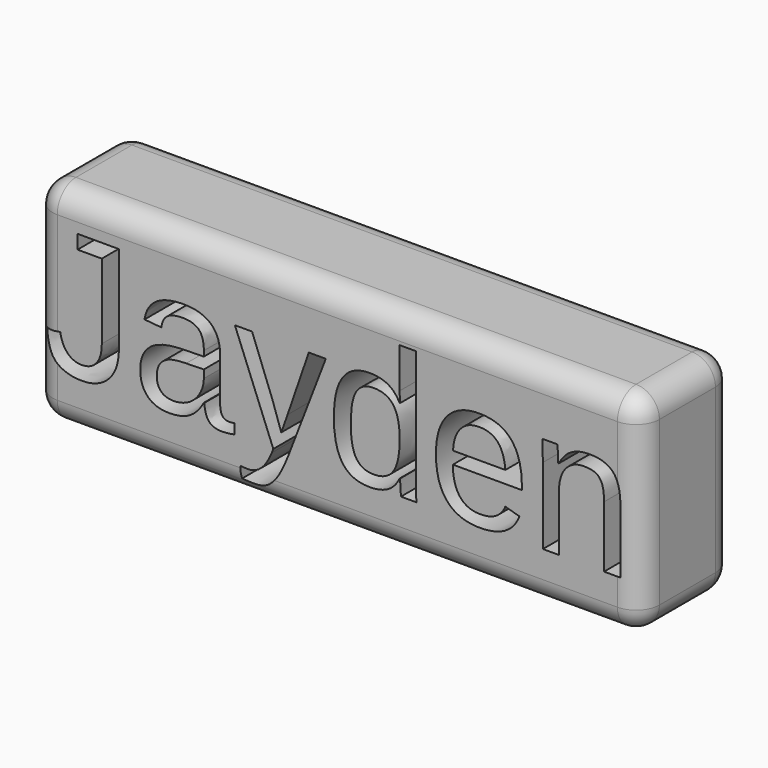
from build123d import *

# Parameters (mm, degrees)
F0_W         = 130
F0_H         = 45
F1_DEPTH     = 25
F2_TEXT_SIZE = 39.2966263462
F3_DEPTH     = 25
F4_T1_DEPTH  = 15
F4_T3_DEPTH  = 35
F4_T5_DEPTH  = 120
F4_S9_W      = 5
F4_S9_H      = 5
F4_T10_DEPTH = 5
F4_S15_W     = 5
F4_S15_H     = 5
F4_T16_DEPTH = 5
F4_S21_W     = 5
F4_S21_H     = 5
F4_T22_DEPTH = 5
F4_S27_W     = 5
F4_S27_H     = 5
F4_T28_DEPTH = 5
F4_S33_W     = 5
F4_S33_H     = 5
F4_T34_DEPTH = 5
F4_S39_W     = 5
F4_S39_H     = 5
F4_T40_DEPTH = 5
F4_S45_W     = 5
F4_S45_H     = 5
F4_T46_DEPTH = 5
F4_S51_W     = 5
F4_S51_H     = 5
F4_T52_DEPTH = 5


# Not quite as in the source:
# - a fillet or chamfer that OpenCascade refuses, or shapes differently, is made with other operations: its cross-section is extruded or revolved along the edge and cut away or added
# - Text() gives the source's letters only with a copy of the font that has no kerning and outlines rounded to 1/6400 em; it was checked with that copy


with BuildPart() as f1:
    # F0 (on Front) → F1 (new body)
    with BuildSketch(Plane.XZ):
        with Locations((65, 22.5)):
            Rectangle(F0_W, F0_H)
    extrude(amount=-F1_DEPTH)

    # F2 (on face) → F3 (cut)
    with BuildSketch(Plane.XZ):
        with Locations((1.4560963027, 10.7717518695)):
            Text('Jayden', F2_TEXT_SIZE, font='Arimo', text_align=(TextAlign.LEFT, TextAlign.BOTTOM))
    extrude(amount=-F3_DEPTH, mode=Mode.SUBTRACT)

    # F4: fillet of radius 5 on 12 edges, made by hand

    # F4_s2 → F4_t1 (cut)
    with BuildSketch(Plane.XZ.offset(-20)):
        with BuildLine():
            ThreePointArc((125, 0), (128.5355339059, 1.4644660941), (130, 5))
            Line((130, 5), (130, 0))
            Line((130, 0), (125, 0))
        make_face()
        with BuildLine():
            ThreePointArc((125, 45), (128.5355339059, 43.5355339059), (130, 40))
            Line((130, 40), (130, 45))
            Line((130, 45), (125, 45))
        make_face()
        with BuildLine():
            ThreePointArc((0, 40), (1.4644660941, 43.5355339059), (5, 45))
            Line((5, 45), (0, 45))
            Line((0, 45), (0, 40))
        make_face()
        with BuildLine():
            ThreePointArc((0, 5), (1.4644660941, 1.4644660941), (5, 0))
            Line((5, 0), (0, 0))
            Line((0, 0), (0, 5))
        make_face()
    extrude(amount=F4_T1_DEPTH, mode=Mode.SUBTRACT)

    # F4_s4 → F4_t3 (cut)
    with BuildSketch(Plane.XY.offset(5)):
        with BuildLine():
            ThreePointArc((125, 0), (128.5355339059, 1.4644660941), (130, 5))
            Line((130, 5), (130, 0))
            Line((130, 0), (125, 0))
        make_face()
        with BuildLine():
            ThreePointArc((125, 25), (128.5355339059, 23.5355339059), (130, 20))
            Line((130, 20), (130, 25))
            Line((130, 25), (125, 25))
        make_face()
        with BuildLine():
            ThreePointArc((0, 5), (1.4644660941, 1.4644660941), (5, 0))
            Line((5, 0), (0, 0))
            Line((0, 0), (0, 5))
        make_face()
        with BuildLine():
            ThreePointArc((0, 20), (1.4644660941, 23.5355339059), (5, 25))
            Line((5, 25), (0, 25))
            Line((0, 25), (0, 20))
        make_face()
    extrude(amount=F4_T3_DEPTH, mode=Mode.SUBTRACT)

    # F4_s6 → F4_t5 (cut)
    with BuildSketch(Plane.YZ.offset(5)):
        with BuildLine():
            ThreePointArc((5, 45), (1.4644660941, 43.5355339059), (0, 40))
            Line((0, 40), (0, 45))
            Line((0, 45), (5, 45))
        make_face()
        with BuildLine():
            ThreePointArc((20, 45), (23.5355339059, 43.5355339059), (25, 40))
            Line((25, 40), (25, 45))
            Line((25, 45), (20, 45))
        make_face()
        with BuildLine():
            ThreePointArc((5, 0), (1.4644660941, 1.4644660941), (0, 5))
            Line((0, 5), (0, 0))
            Line((0, 0), (5, 0))
        make_face()
        with BuildLine():
            ThreePointArc((20, 0), (23.5355339059, 1.4644660941), (25, 5))
            Line((25, 5), (25, 0))
            Line((25, 0), (20, 0))
        make_face()
    extrude(amount=F4_T5_DEPTH, mode=Mode.SUBTRACT)


with BuildPart() as f4_tool8:
    # F4_s9 → F4_t10 (new body)
    with BuildSketch(Plane.XY.offset(5)):
        with Locations((127.5, 2.5)):
            Rectangle(F4_S9_W, F4_S9_H)
    extrude(amount=-F4_T10_DEPTH)

    # F4_s11 → F4_t12 (revolve, cut)
    with BuildSketch(Plane(origin=(125, 5, 5), x_dir=(-0.7071067812, 0.7071067812, 0), z_dir=(-0.7071067812, -0.7071067812, 0))):
        with BuildLine():
            ThreePointArc((0, -5), (5, 0), (0, 5))
            Line((0, 5), (0, -5))
        make_face()
    revolve(axis=Axis((125, 5, 5), (0, 0, -1)), mode=Mode.SUBTRACT)


with BuildPart() as f1_1:
    add(f1.part)

    # F4_t7: cut F4_tool8
    add(f4_tool8.part, mode=Mode.SUBTRACT)


with BuildPart() as f4_tool14:
    # F4_s15 → F4_t16 (new body)
    with BuildSketch(Plane.XY.offset(5)):
        with Locations((127.5, 22.5)):
            Rectangle(F4_S15_W, F4_S15_H)
    extrude(amount=-F4_T16_DEPTH)

    # F4_s17 → F4_t18 (revolve, cut)
    with BuildSketch(Plane(origin=(125, 20, 5), x_dir=(-0.7071067812, -0.7071067812, 0), z_dir=(0.7071067812, -0.7071067812, 0))):
        with BuildLine():
            ThreePointArc((0, -5), (5, 0), (0, 5))
            Line((0, 5), (0, -5))
        make_face()
    revolve(axis=Axis((125, 20, 5), (0, 0, -1)), mode=Mode.SUBTRACT)


with BuildPart() as f1_2:
    add(f1_1.part)

    # F4_t13: cut F4_tool14
    add(f4_tool14.part, mode=Mode.SUBTRACT)


with BuildPart() as f4_tool20:
    # F4_s21 → F4_t22 (new body)
    with BuildSketch(Plane.XY.offset(40)):
        with Locations((127.5, 2.5)):
            Rectangle(F4_S21_W, F4_S21_H)
    extrude(amount=F4_T22_DEPTH)

    # F4_s23 → F4_t24 (revolve, cut)
    with BuildSketch(Plane(origin=(125, 5, 40), x_dir=(-0.7071067812, 0.7071067812, 0), z_dir=(0.7071067812, 0.7071067812, 0))):
        with BuildLine():
            ThreePointArc((0, -5), (5, 0), (0, 5))
            Line((0, 5), (0, -5))
        make_face()
    revolve(axis=Axis((125, 5, 40), (0, 0, 1)), mode=Mode.SUBTRACT)


with BuildPart() as f1_3:
    add(f1_2.part)

    # F4_t19: cut F4_tool20
    add(f4_tool20.part, mode=Mode.SUBTRACT)


with BuildPart() as f4_tool26:
    # F4_s27 → F4_t28 (new body)
    with BuildSketch(Plane.XY.offset(40)):
        with Locations((127.5, 22.5)):
            Rectangle(F4_S27_W, F4_S27_H)
    extrude(amount=F4_T28_DEPTH)

    # F4_s29 → F4_t30 (revolve, cut)
    with BuildSketch(Plane(origin=(125, 20, 40), x_dir=(-0.7071067812, -0.7071067812, 0), z_dir=(-0.7071067812, 0.7071067812, 0))):
        with BuildLine():
            ThreePointArc((0, -5), (5, 0), (0, 5))
            Line((0, 5), (0, -5))
        make_face()
    revolve(axis=Axis((125, 20, 40), (0, 0, 1)), mode=Mode.SUBTRACT)


with BuildPart() as f1_4:
    add(f1_3.part)

    # F4_t25: cut F4_tool26
    add(f4_tool26.part, mode=Mode.SUBTRACT)


with BuildPart() as f4_tool32:
    # F4_s33 → F4_t34 (new body)
    with BuildSketch(Plane.YZ.offset(5)):
        with Locations((2.5, 42.5)):
            Rectangle(F4_S33_W, F4_S33_H)
    extrude(amount=-F4_T34_DEPTH)

    # F4_s35 → F4_t36 (revolve, cut)
    with BuildSketch(Plane(origin=(5, 5, 40), x_dir=(0, 0.7071067812, -0.7071067812), z_dir=(0, 0.7071067812, 0.7071067812))):
        with BuildLine():
            ThreePointArc((0, -5), (5, 0), (0, 5))
            Line((0, 5), (0, -5))
        make_face()
    revolve(axis=Axis((5, 5, 40), (-1, 0, 0)), mode=Mode.SUBTRACT)


with BuildPart() as f1_5:
    add(f1_4.part)

    # F4_t31: cut F4_tool32
    add(f4_tool32.part, mode=Mode.SUBTRACT)


with BuildPart() as f4_tool38:
    # F4_s39 → F4_t40 (new body)
    with BuildSketch(Plane.YZ.offset(5)):
        with Locations((22.5, 42.5)):
            Rectangle(F4_S39_W, F4_S39_H)
    extrude(amount=-F4_T40_DEPTH)

    # F4_s41 → F4_t42 (revolve, cut)
    with BuildSketch(Plane(origin=(5, 20, 40), x_dir=(0, -0.7071067812, -0.7071067812), z_dir=(0, 0.7071067812, -0.7071067812))):
        with BuildLine():
            ThreePointArc((0, -5), (5, 0), (0, 5))
            Line((0, 5), (0, -5))
        make_face()
    revolve(axis=Axis((5, 20, 40), (-1, 0, 0)), mode=Mode.SUBTRACT)


with BuildPart() as f1_6:
    add(f1_5.part)

    # F4_t37: cut F4_tool38
    add(f4_tool38.part, mode=Mode.SUBTRACT)


with BuildPart() as f4_tool44:
    # F4_s45 → F4_t46 (new body)
    with BuildSketch(Plane.YZ.offset(5)):
        with Locations((2.5, 2.5)):
            Rectangle(F4_S45_W, F4_S45_H)
    extrude(amount=-F4_T46_DEPTH)

    # F4_s47 → F4_t48 (revolve, cut)
    with BuildSketch(Plane(origin=(5, 5, 5), x_dir=(0, 0.7071067812, 0.7071067812), z_dir=(0, -0.7071067812, 0.7071067812))):
        with BuildLine():
            ThreePointArc((0, -5), (5, 0), (0, 5))
            Line((0, 5), (0, -5))
        make_face()
    revolve(axis=Axis((5, 5, 5), (-1, 0, 0)), mode=Mode.SUBTRACT)


with BuildPart() as f1_7:
    add(f1_6.part)

    # F4_t43: cut F4_tool44
    add(f4_tool44.part, mode=Mode.SUBTRACT)


with BuildPart() as f4_tool50:
    # F4_s51 → F4_t52 (new body)
    with BuildSketch(Plane.YZ.offset(5)):
        with Locations((22.5, 2.5)):
            Rectangle(F4_S51_W, F4_S51_H)
    extrude(amount=-F4_T52_DEPTH)

    # F4_s53 → F4_t54 (revolve, cut)
    with BuildSketch(Plane(origin=(5, 20, 5), x_dir=(0, -0.7071067812, 0.7071067812), z_dir=(0, -0.7071067812, -0.7071067812))):
        with BuildLine():
            ThreePointArc((0, -5), (5, 0), (0, 5))
            Line((0, 5), (0, -5))
        make_face()
    revolve(axis=Axis((5, 20, 5), (-1, 0, 0)), mode=Mode.SUBTRACT)


with BuildPart() as f1_8:
    add(f1_7.part)

    # F4_t49: cut F4_tool50
    add(f4_tool50.part, mode=Mode.SUBTRACT)


solid = f1_8.part
